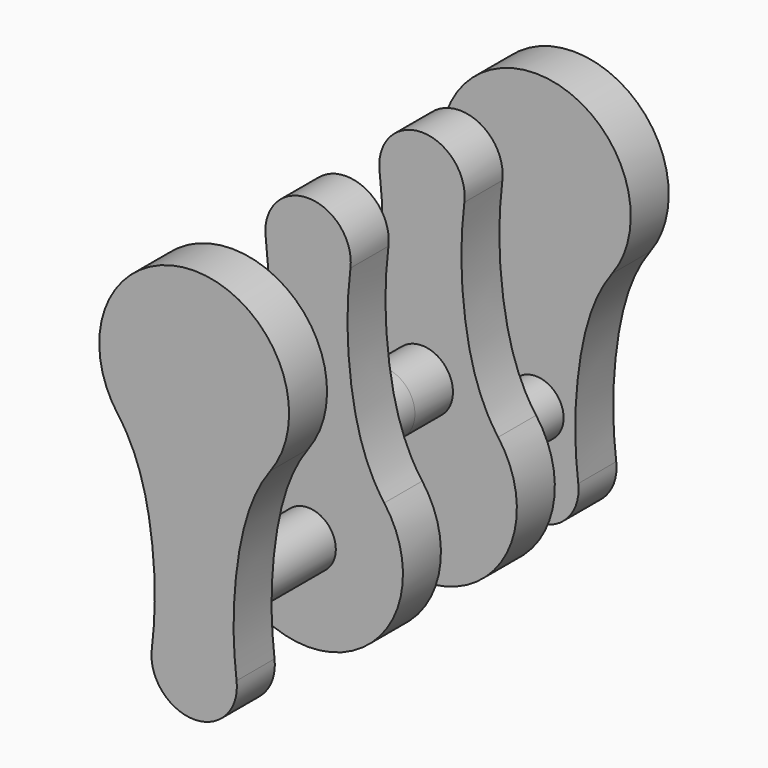
from build123d import *

# Parameters (mm, degrees)
F1_DEPTH = 25.4
F2_R     = 14.8583693586
F3_DEPTH = 50.8
F5_DEPTH = 25.4
F6_R     = 16.5750816165
F7_DEPTH = 25.4


# Not quite as in the source:
# - the dataset's text gives a spline's control points without its knots; the knots are read off the source's solid


with BuildPart() as f1:
    # F0 (on Front) → F1 (new body)
    with BuildSketch(Plane.XZ):
        with BuildLine():
            add(Edge.make_bspline(
                [(-22.6914668872, 135.0717148125), (-20.5500892533, 117.5344431572), (-20.5383703228, 83.7697737674), (-29.499421348, 45.4828893303), (-40.7842174417, 30.2867563082)],
                knots=[0, 0, 0, 0, 0.4898289436, 1, 1, 1, 1], degree=3))
            ThreePointArc((-40.7842174417, 30.2867563082), (0, -50.8), (40.7842174417, 30.2867563082))
            add(Edge.make_bspline(
                [(22.6914668872, 135.0717148125), (20.5500892533, 117.5344431572), (20.5383703228, 83.7697737674), (29.499421348, 45.4828893303), (40.7842174417, 30.2867563082)],
                knots=[0, 0, 0, 0, 0.4898289436, 1, 1, 1, 1], degree=3))
            ThreePointArc((22.6914668872, 135.0717148125), (0, 160.7024422453), (-22.6914668872, 135.0717148125))
        make_face()
    extrude(amount=F1_DEPTH)

    # F2 (on face) → F3 (join)
    with BuildSketch(Plane.XZ.offset(25.4)):
        Circle(F2_R)
    extrude(amount=F3_DEPTH)

    # F4 (on face) → F5 (join)
    with BuildSketch(Plane.XZ.offset(76.2)):
        with BuildLine():
            ThreePointArc((40.7842174417, 76.3932436918), (0, 157.48), (-40.7842174417, 76.3932436918))
            add(Edge.make_bspline(
                [(-29.0914526999, 53.34), (-31.8632962455, 61.5801736989), (-35.6211262818, 69.4406129646), (-40.7842174417, 76.3932436918)],
                knots=[0.7665833171, 0.7665833171, 0.7665833171, 0.7665833171, 1, 1, 1, 1], degree=3))
            add(Edge.make_bspline(
                [(-29.0914526999, 53.34), (-25.8049702839, 43.5699009594), (-20.5411057167, 15.0289891053), (-20.5500892533, -10.8544431572), (-22.6914668872, -28.3917148125)],
                knots=[0.2334166829, 0.2334166829, 0.2334166829, 0.2334166829, 0.5101710564, 1, 1, 1, 1], degree=3))
            ThreePointArc((-22.6914668872, -28.3917148125), (0, -54.0224422453), (22.6914668872, -28.3917148125))
            add(Edge.make_bspline(
                [(40.7842174417, 76.3932436918), (29.499421348, 61.1971106697), (20.5383703228, 22.9102262326), (20.5500892533, -10.8544431572), (22.6914668872, -28.3917148125)],
                knots=[0, 0, 0, 0, 0.5101710564, 1, 1, 1, 1], degree=3))
        make_face()
    extrude(amount=F5_DEPTH)

    # F6 (on face) → F7 (join)
    with BuildSketch(Plane(origin=(0, 0, 0), x_dir=(-1, 0, 0), z_dir=(0, 1, 0))):
        with Locations((0, 43.6854362488)):
            Circle(F6_R)
    extrude(amount=F7_DEPTH)

    # F8: F1 across face


with BuildPart() as f1_1:
    add(f1.part)
    add(f1.part.mirror(Plane(origin=(0, 25.4, 43.6854362488), x_dir=(-1, 0, 0), z_dir=(0, 1, 0))))


solid = f1_1.part
